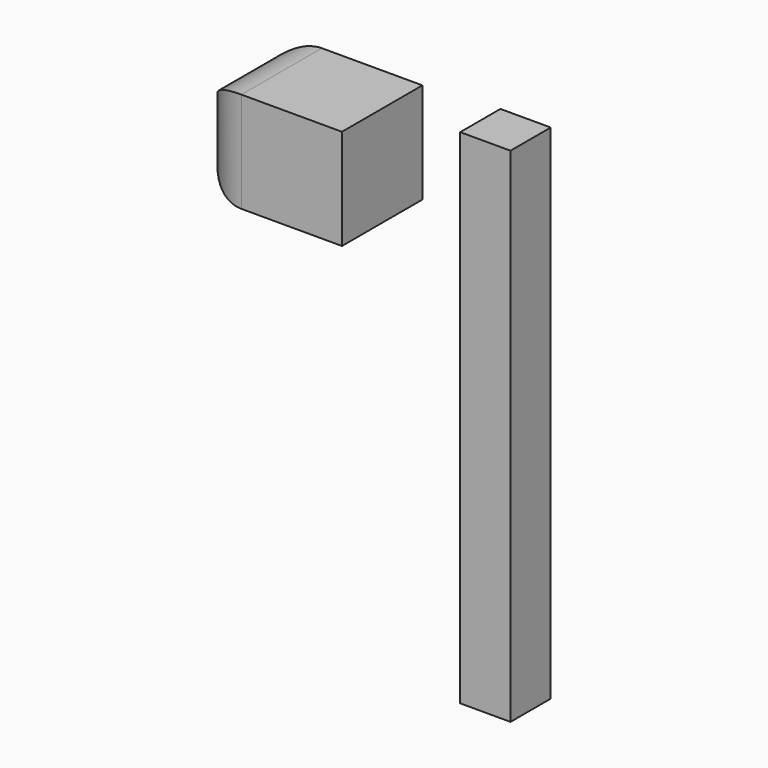
from build123d import *

# Parameters (mm, degrees)
F0_W     = 10
F0_H     = 100
F1_DEPTH = 10
F2_W     = 30
F2_H     = 20
F3_DEPTH = 20
F4_R     = 9.99999


# Not quite as in the source:
# - a fillet or chamfer is up to 0.001 mm smaller than in the source, because OpenCascade refuses the exact size


with BuildPart() as f1:
    # F0 (on Front) → F1 (new body)
    with BuildSketch(Plane.XZ):
        with Locations((-5.3346473165, -12.30174932)):
            Rectangle(F0_W, F0_H)
    extrude(amount=F1_DEPTH)


with BuildPart() as f3:
    # F2 (on Front) → F3 (new body)
    with BuildSketch(Plane.XZ):
        with Locations((-40.8489312977, 26.7800622059)):
            Rectangle(F2_W, F2_H)
    extrude(amount=F3_DEPTH)

    # F4 (radius 10 in the source; OpenCascade refuses exactly that, so slightly less here)
    f4_edges = [f3.edges().sort_by_distance(p)[0] for p in [
        (-55.848931, -10, 36.780062),
        (-55.848931, -10, 16.780062),
        (-55.848931, 0, 26.780062),
        (-55.848931, -20, 26.780062),
    ]]
    fillet(f4_edges, radius=F4_R)


solid = Compound([f1.part, f3.part])
